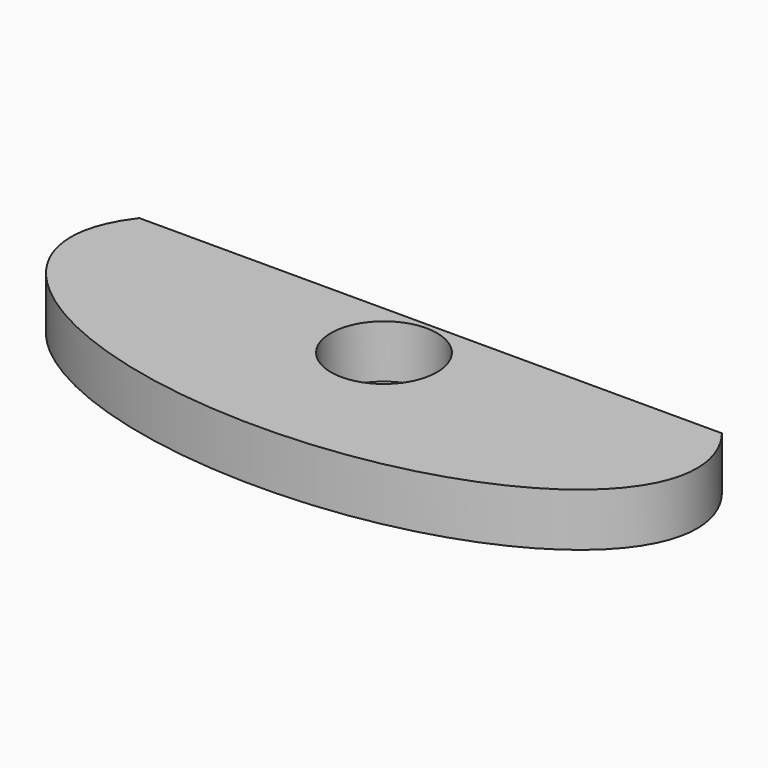
from build123d import *

# Parameters (mm, degrees)
F1_DEPTH = 5
F2_R     = 5
F3_DEPTH = 25
F5_DEPTH = 25


# Not quite as in the source:
# - a feature names something its author has since deleted; it is built from what else it names


with BuildPart() as f1:
    # F0 (on Top) → F1 (new body)
    with BuildSketch(Plane.XY):
        with BuildLine():
            add(Edge.make_bspline(
                [(-66.2264598608, 20.3643515706), (-66.2264598608, -5.6164105429), (-21.9764598608, 7.3739705138), (22.2735401392, 20.3643515706), (-21.9764598608, 33.3547326274), (-66.2264598608, 46.3451136841), (-66.2264598608, 20.3643515706)],
                knots=[0, 0, 0, 2.0943951024, 2.0943951024, 4.1887902048, 4.1887902048, 6.2831853072, 6.2831853072, 6.2831853072], degree=2, weights=[1, 0.5, 1, 0.5, 1, 0.5, 1]))
        make_face()
    extrude(amount=F1_DEPTH)

    # F2 (on face) → F3 (cut)
    with BuildSketch(Plane.XY.offset(5)):
        with Locations((-36.7264598608, 20.3643515706)):
            Circle(F2_R)
    extrude(amount=-F3_DEPTH, mode=Mode.SUBTRACT)

    # F4 (on face) → F5 (cut)
    with BuildSketch(Plane.XY.offset(5)):
        with BuildLine():
            add(Edge.make_bspline(
                [(-9.2786523325, 25.8612383577), (-13.0541377648, 30.7354249678), (-21.9764598608, 33.3547326274), (-51.6274393448, 42.0593094003), (-64.1742673891, 25.8612383577)],
                knots=[3.4859107004, 3.4859107004, 3.4859107004, 4.1887902048, 4.1887902048, 5.8694408983, 5.8694408983, 5.8694408983], degree=2, weights=[0.7770272803, 0.8321998787, 1, 0.5987742018, 0.8414769682]))
            Line((-64.1742673891, 25.8612383577), (-9.2786523325, 25.8612383577))
        make_face()
    extrude(amount=-F5_DEPTH, mode=Mode.SUBTRACT)


solid = f1.part
